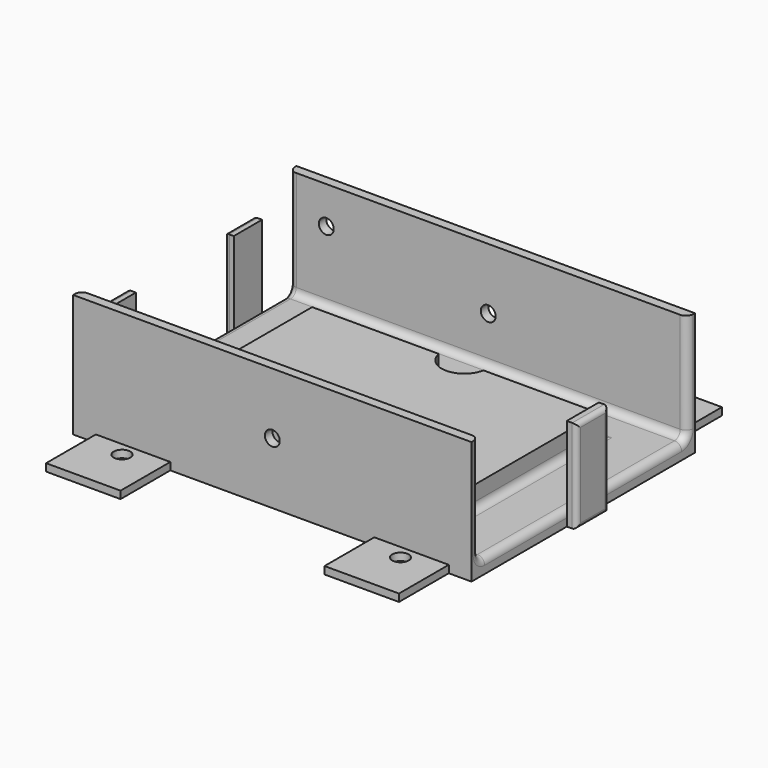
from build123d import *

# Parameters (mm, degrees)
F1_DEPTH  = 4
F0_W      = 107
F0_H      = 2.5
F2_DEPTH  = 33
F3_W      = 20
F3_H      = 19.215
F3_R      = 2.2232187412
F4_DEPTH  = 2
F6_D      = 4
F6_DEPTH  = 12
F6_TIP    = 1.2017212381
F7_D      = 4
F8_DEPTH  = 10
F9_F1_R   = 1.9313708499
F9_F2_R   = 1.9313708499
F10_W     = 15
F10_H     = 10
F11_DEPTH = 11.3
F0_W_2    = 2.4193752706
F0_H_2    = 9.5048956573
F0_W_3    = 2.649404496
F0_H_3    = 10.744664818
F12_DEPTH = 25
F13_R     = 1.2071067812


with BuildPart() as f1:
    # F0 (on Top) → F1 (new body)
    with BuildSketch(Plane.XY):
        Polygon((-53.5, -35), (53.5, -35), (53.5, -5.4848068394), (53.5, 5.2598579787), (53.5, 35), (-53.5, 35), (-53.5, 25.9394217283), (-53.5, 16.434526071), (-53.5, -16.434526071), (-53.5, -25.9394217283), align=None)
        with BuildLine():
            Line((38.5, 24), (38.5, -24))
            Line((38.5, -24), (7.5, -24))
            ThreePointArc((7.5, -24), (1.5, -19), (-4.5, -24))
            Line((-4.5, -24), (-38.5, -24))
            Line((-38.5, -24), (-38.5, 24))
            Line((-38.5, 24), (-4.5, 24))
            ThreePointArc((-4.5, 24), (1.5, 19), (7.5, 24))
            Line((7.5, 24), (38.5, 24))
        make_face(mode=Mode.SUBTRACT)
    extrude(amount=F1_DEPTH)

    # F0 (on Top) → F2 (join)
    with BuildSketch(Plane.XY):
        with Locations((0, 36.25)):
            Rectangle(F0_W, F0_H)
        with Locations((0, -36.25)):
            Rectangle(F0_W, F0_H)
    extrude(amount=F2_DEPTH)

    # F3 (on face) → F4 (join)
    with BuildSketch(Plane.XY):
        with Locations((-37.3952314258, -44.6075)):
            Rectangle(F3_W, F3_H)
        with Locations((-37.3952314258, -41.215)):
            Circle(F3_R, mode=Mode.SUBTRACT)
        with Locations((37.3952314258, -44.6075)):
            Rectangle(F3_W, F3_H)
        with Locations((37.3952314258, -41.215)):
            Circle(F3_R, mode=Mode.SUBTRACT)
        with Locations((37.3952314258, 44.6075)):
            Rectangle(F3_W, F3_H)
        with Locations((37.3952314258, 41.215)):
            Circle(F3_R, mode=Mode.SUBTRACT)
        with Locations((-37.3952314258, 44.6075)):
            Rectangle(F3_W, F3_H)
        with Locations((-37.3952314258, 41.215)):
            Circle(F3_R, mode=Mode.SUBTRACT)
    extrude(amount=F4_DEPTH)

    # F6
    with Locations(Plane(origin=(0, 37.5, 0), x_dir=(-1, 0, 0), z_dir=(0, 1, 0))):
        with Locations((43.5, 23)):
            Hole(F6_D / 2, depth=F6_DEPTH)
            with Locations((0, 0, -(F6_DEPTH + F6_TIP / 2))):  # 118° drill point
                Cone(0, F6_D / 2, F6_TIP, mode=Mode.SUBTRACT)

    # F7 (through all)
    with Locations(Plane(origin=(0, 37.5, 0), x_dir=(-1, 0, 0), z_dir=(0, 1, 0))):
        with Locations((0, 16.522007063)):
            Hole(F7_D / 2)

    # F0 (on Top) → F8 (join)
    with BuildSketch(Plane.XY):
        with BuildLine():
            Line((7.5, -24), (38.5, -24))
            Line((38.5, -24), (38.5, 24))
            Line((38.5, 24), (7.5, 24))
            ThreePointArc((7.5, 24), (1.5, 19), (-4.5, 24))
            Line((-4.5, 24), (-38.5, 24))
            Line((-38.5, 24), (-38.5, -24))
            Line((-38.5, -24), (-4.5, -24))
            ThreePointArc((-4.5, -24), (1.5, -19), (7.5, -24))
        make_face()
    extrude(amount=F8_DEPTH)

    # F9: fillet of radius 1.9313708499 on 12 edges, made by hand

    # F9_f1
    f9_f1_edges = [f1.edges().sort_by_distance(p)[0] for p in [
        (0, -35, 4),
        (0, 35, 4),
        (1.5, 19, 4),
        (23, 24, 4),
        (38.5, 0, 4),
        (23, -24, 4),
        (1.5, -19, 4),
        (-21.5, -24, 4),
        (-38.5, 0, 4),
        (-21.5, 24, 4),
    ]]
    fillet(f9_f1_edges, radius=F9_F1_R)

    # F9_f2
    f9_f2_edges = [f1.edges().sort_by_distance(p)[0] for p in [
        (53.5, 0, 4),
        (-53.5, 0, 4),
        (-53.5, -34.4343145751, 4.5656854249),
        (-53.5, 34.4343145751, 4.5656854249),
        (53.5, 34.4343145751, 4.5656854249),
        (53.5, -34.4343145751, 4.5656854249),
    ]]
    fillet(f9_f2_edges, radius=F9_F2_R)

    # F10 (on face) → F11 (cut)
    with BuildSketch(Plane.XY):
        with Locations((-46.3137403131, 0)):
            Rectangle(F10_W, F10_H)
    extrude(amount=F11_DEPTH, mode=Mode.SUBTRACT)

    # F0 (on Top) → F12 (join)
    with BuildSketch(Plane.XY):
        with Locations((-54.7096876353, 21.1869738996)):
            Rectangle(F0_W_2, F0_H_2)
        with Locations((-54.7096876353, -21.1869738996)):
            Rectangle(F0_W_2, F0_H_2)
        with Locations((54.824702248, -0.1124744304)):
            Rectangle(F0_W_3, F0_H_3)
    extrude(amount=F12_DEPTH)

    # F13
    f13_edges = [f1.edges().sort_by_distance(p)[0] for p in [
        (-55.919375, 25.939422, 12.5),
        (-55.919375, 16.434526, 12.5),
        (-55.919375, 21.186974, 0),
        (-55.919375, 21.186974, 25),
        (-55.919375, -16.434526, 12.5),
        (-55.919375, -25.939422, 12.5),
        (-55.919375, -21.186974, 0),
        (-55.919375, -21.186974, 25),
        (56.149404, -5.484807, 12.5),
        (56.149404, 5.259858, 12.5),
        (56.149404, -0.112474, 0),
        (56.149404, -0.112474, 25),
    ]]
    fillet(f13_edges, radius=F13_R)


solid = f1.part
